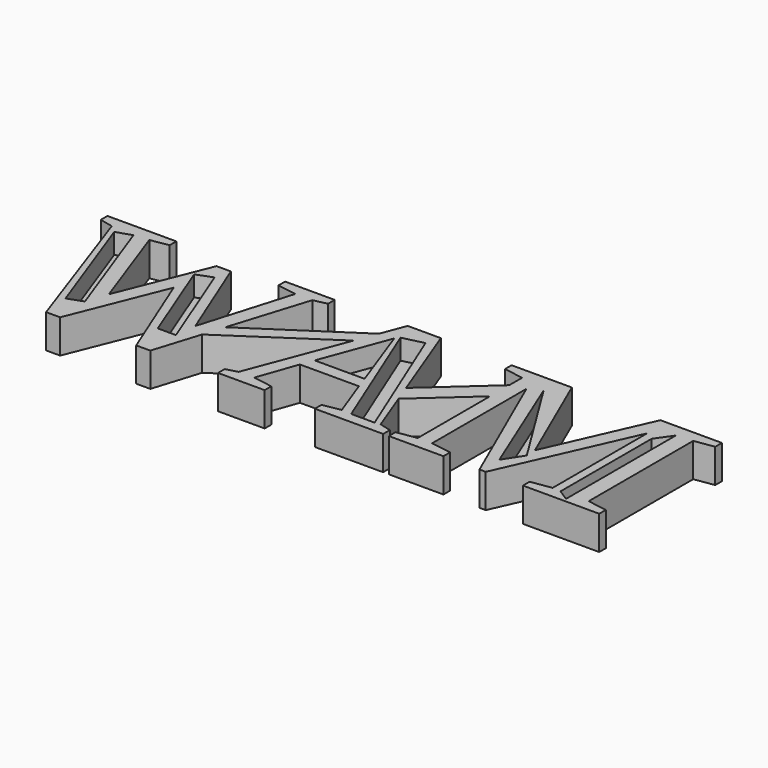
from build123d import *

# Parameters (mm, degrees)
F1_DEPTH = 5
F2_DEPTH = 2


with BuildPart() as f1:
    # F0 (on Top) → F1 (new body)
    with BuildSketch(Plane.XY):
        Polygon((-19.2634474565, -6.1269301263), (-18.2925394874, -3.0197121847), (-14.6755642361, 8.5557725694), (-12.6898871528, 9.0006510417), (-12.6898871528, 10.2376302083), (-20.0466579861, 10.2376302083), (-20.0466579861, 9.0006510417), (-17.1820746528, 8.5557725694), (-21.2022569444, -4.9533420139), (-26.5407986111, 8.30078125), (-28.662109375, 8.30078125), (-33.984375, -4.9913194444), (-38.8346354167, 8.5557725694), (-36.1707899306, 9.0006510417), (-36.1707899306, 10.2376302083), (-46.3758680556, 10.2376302083), (-46.3758680556, 9.0006510417), (-44.3956163194, 8.5557725694), (-36.865234375, -13.0262586806), (-34.7819010417, -13.0262586806), (-29.1666666667, 0.9982638889), (-23.5080295139, -13.0262586806), (-21.4192708333, -13.0262586806), align=None)
        Polygon((-43.2690681627, 7.6009020128), (-41.0144999623, 8.3526074886), (-35.0183658302, -8.1367557868), (-37.251050357, -8.9486413444), align=None, mode=Mode.SUBTRACT)
        Polygon((-29.3969921768, 5.0547351129), (-27.0734913647, 5.9541547671), (-21.5270686895, -8.1367557868), (-24.2253281176, -8.1367557868), align=None, mode=Mode.SUBTRACT)
        Polygon((-4.6070118818, 3.644027612), (-3.3984823364, 6.814897888), (-18.2925394874, -3.0197121847), (-19.2634474565, -6.1269301263), align=None)
        Polygon((-2.0236545139, 10.4220920139), (-3.3984823364, 6.814897888), (-4.6070118818, 3.644027612), (-10.1128472222, -10.8018663194), (-11.8055555556, -11.2630208333), (-11.8055555556, -12.5), (-4.8882378472, -12.5), (-4.8882378472, -11.2630208333), (-7.8070746528, -10.8018663194), (-5.7237413194, -4.9207899306), (3.0110677083, -4.9207899306), (5.1812065972, -10.8018663194), (2.5499131944, -11.2630208333), (2.5499131944, -12.5), (12.6736111111, -12.5), (12.6736111111, -11.2630208333), (10.9429253472, -10.8018663194), (8.5519227834, -4.4988999923), (7.5429662144, -1.8391708158), (2.8917100694, 10.4220920139), align=None)
        Polygon((-5.0238715278, -3.0544704861), (-1.2803819444, 6.9986979167), (2.3654513889, -3.0544704861), align=None, mode=Mode.SUBTRACT)
        Polygon((-0.8333516307, 7.6009020128), (2.2724873852, 8.3526074886), (10.1284366101, -10.9029943123), (6.6572050564, -10.9029943123), align=None, mode=Mode.SUBTRACT)
        Polygon((16.4388020833, 6.1594187407), (7.5429662144, -1.8391708158), (8.5519227834, -4.4988999923), (16.4388020833, 2.5924977505), align=None)
        Polygon((16.4388020833, 8.5557725694), (16.4388020833, 6.1594187407), (16.4388020833, 2.5924977505), (16.4388020833, -10.8018663194), (13.5199652778, -11.2630208333), (13.5199652778, -12.5), (21.6091579861, -12.5), (21.6091579861, -11.2630208333), (18.5601128472, -10.8018663194), (18.5601128472, 6.7111545139), (26.9476996528, -12.5), (27.880859375, -12.5), (36.4420572917, 6.7111545139), (36.4420572917, -10.8018663194), (33.3930121528, -11.2630208333), (33.3930121528, -12.5), (44.6994357639, -12.5), (44.6994357639, -11.2630208333), (41.7860243056, -10.8018663194), (41.7860243056, 8.5557725694), (44.6994357639, 9.0006510417), (44.6994357639, 10.2376302083), (35.5794270833, 10.2376302083), (28.9496527778, -4.7200520833), (22.4555121528, 10.2376302083), (13.5199652778, 10.2376302083), (13.5199652778, 9.0006510417), align=None)
        Polygon((37.6935936511, -10.9029943123), (37.6935936511, 5.9541547671), (39.3697134069, 8.3526074886), (39.3697134069, -11.9900868907), align=None, mode=Mode.SUBTRACT)
        Polygon((27.211471604, -9.1471979388), (20.3785393387, 7.6009020128), (29.0340669453, -6.3370526768), align=None, mode=Mode.SUBTRACT)
    extrude(amount=F1_DEPTH)

    # F0 (on Top) → F2 (join)
    with BuildSketch(Plane.XY):
        Polygon((-21.5270686895, -8.1367557868), (-27.0734913647, 5.9541547671), (-29.3969921768, 5.0547351129), (-24.2253281176, -8.1367557868), align=None)
        Polygon((-35.0183658302, -8.1367557868), (-41.0144999623, 8.3526074886), (-43.2690681627, 7.6009020128), (-37.251050357, -8.9486413444), align=None)
        Polygon((10.1284366101, -10.9029943123), (2.2724873852, 8.3526074886), (-0.8333516307, 7.6009020128), (6.6572050564, -10.9029943123), align=None)
        Polygon((2.3654513889, -3.0544704861), (-1.2803819444, 6.9986979167), (-5.0238715278, -3.0544704861), align=None)
        Polygon((29.0340669453, -6.3370526768), (20.3785393387, 7.6009020128), (27.211471604, -9.1471979388), align=None)
        Polygon((39.3697134069, 8.3526074886), (37.6935936511, 5.9541547671), (37.6935936511, -10.9029943123), (39.3697134069, -11.9900868907), align=None)
    extrude(amount=F2_DEPTH)


solid = f1.part
